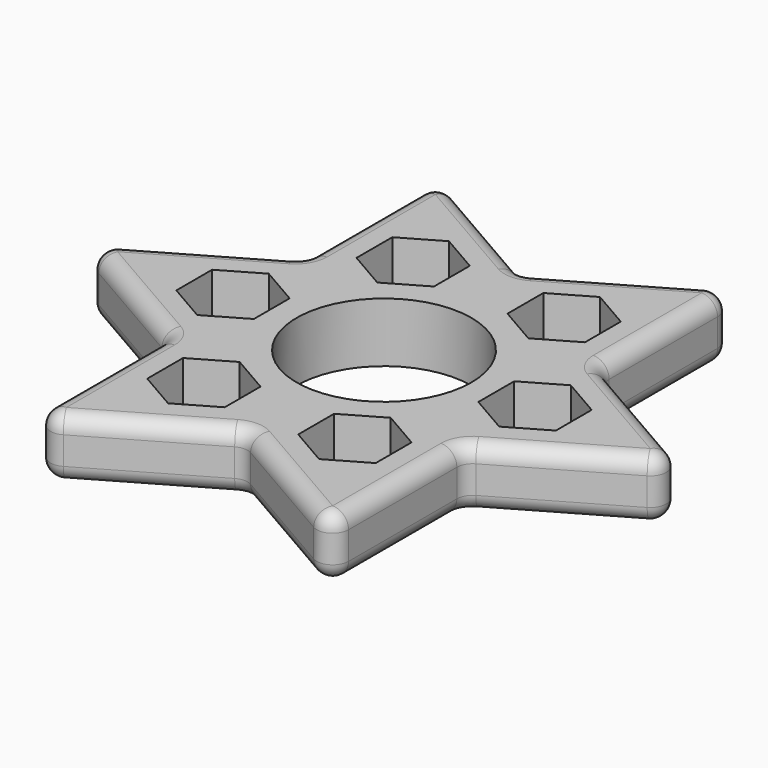
from build123d import *

# Parameters (mm, degrees)
F0_R            = 11
F1_DEPTH        = 7.5
F2_R            = 2
F3_R            = 2
F5_DEPTH        = 25
F5_COPIES_COUNT = 6


# Not quite as in the source:
# - a pattern or mirror of a feature is missing from the dataset's text; its kind, count and spacing are read off the source's solid


with BuildPart() as f1:
    # F0 (on Top) → F1 (new body)
    with BuildSketch(Plane.XY):
        Polygon((0, 21.6506350946), (-18.75, 32.4759526419), (-18.75, 10.8253175473), align=None)
        Polygon((0, 21.6506350946), (-18.75, 10.8253175473), (-18.75, -10.8253175473), (0, -21.6506350946), (18.75, -10.8253175473), (18.75, 10.8253175473), align=None)
        Circle(F0_R, mode=Mode.SUBTRACT)
        Polygon((-18.75, -10.8253175473), (-18.75, 10.8253175473), (-37.5, 0), align=None)
        Polygon((18.75, 32.4759526419), (0, 21.6506350946), (18.75, 10.8253175473), align=None)
        Polygon((0, -21.6506350946), (-18.75, -10.8253175473), (-18.75, -32.4759526419), align=None)
        Polygon((37.5, 0), (18.75, 10.8253175473), (18.75, -10.8253175473), align=None)
        Polygon((18.75, -10.8253175473), (0, -21.6506350946), (18.75, -32.4759526419), align=None)
    extrude(amount=F1_DEPTH)

    # F2
    f2_edges = [f1.edges().sort_by_distance(p)[0] for p in [
        (-18.75, -32.475953, 3.75),
        (0, -21.650635, 3.75),
        (18.75, -32.475953, 3.75),
        (18.75, -10.825318, 3.75),
        (37.5, 0, 3.75),
        (18.75, 10.825318, 3.75),
        (18.75, 32.475953, 3.75),
        (0, 21.650635, 3.75),
        (-18.75, 32.475953, 3.75),
        (-37.5, 0, 3.75),
        (-18.75, -10.825318, 3.75),
        (-18.75, 10.825318, 3.75),
    ]]
    fillet(f2_edges, radius=F2_R)

    # F3
    f3_edges = [f1.edges().sort_by_distance(p)[0] for p in [
        (-8.375, -26.485944, 0),
        (-8.375, -26.485944, 7.5),
        (-18.75, 20.495935, 0),
        (-18.75, 20.495935, 7.5),
        (-17.75, 30.743902, 0),
        (-19.017949, 10.980018, 0),
        (-8.375, 26.485944, 0),
        (-27.125, 5.990009, 0),
        (0, 21.960036, 0),
        (-35.5, 0, 0),
        (8.375, 26.485944, 0),
        (-27.125, -5.990009, 0),
        (17.75, 30.743902, 0),
        (-19.017949, -10.980018, 0),
        (18.75, 20.495935, 0),
        (-18.75, -20.495935, 0),
        (19.017949, 10.980018, 0),
        (-17.75, -30.743902, 0),
        (27.125, 5.990009, 0),
        (35.5, 0, 0),
        (0, -21.960036, 0),
        (27.125, -5.990009, 0),
        (8.375, -26.485944, 0),
        (19.017949, -10.980018, 0),
        (17.75, -30.743902, 0),
        (18.75, -20.495935, 0),
        (-17.75, 30.743902, 7.5),
        (-19.017949, 10.980018, 7.5),
        (-8.375, 26.485944, 7.5),
        (-27.125, 5.990009, 7.5),
        (0, 21.960036, 7.5),
        (-35.5, 0, 7.5),
        (8.375, 26.485944, 7.5),
        (-27.125, -5.990009, 7.5),
        (17.75, 30.743902, 7.5),
        (-19.017949, -10.980018, 7.5),
        (18.75, 20.495935, 7.5),
        (-18.75, -20.495935, 7.5),
        (19.017949, 10.980018, 7.5),
        (-17.75, -30.743902, 7.5),
        (27.125, 5.990009, 7.5),
        (35.5, 0, 7.5),
        (0, -21.960036, 7.5),
        (27.125, -5.990009, 7.5),
        (8.375, -26.485944, 7.5),
        (19.017949, -10.980018, 7.5),
        (17.75, -30.743902, 7.5),
        (18.75, -20.495935, 7.5),
    ]]
    fillet(f3_edges, radius=F3_R)

    # F4 (on face) → F5 (cut)
    with BuildSketch(Plane.XY.offset(7.5)):
        Polygon((-14.125, -2.8145825623), (-14.125, 2.8145825623), (-19, 5.6291651246), (-23.875, 2.8145825623), (-23.875, -2.8145825623), (-19, -5.6291651246), align=None)
    f5 = extrude(amount=-F5_DEPTH, mode=Mode.SUBTRACT)

    # F5_copies: F5 ×6 about axis
    f5_copies_axis = Axis((0, 0, 0), (0, 0, 1))
    for i in range(1, F5_COPIES_COUNT):
        add(f5.rotate(f5_copies_axis, i * 360 / F5_COPIES_COUNT), mode=Mode.SUBTRACT)


solid = f1.part
